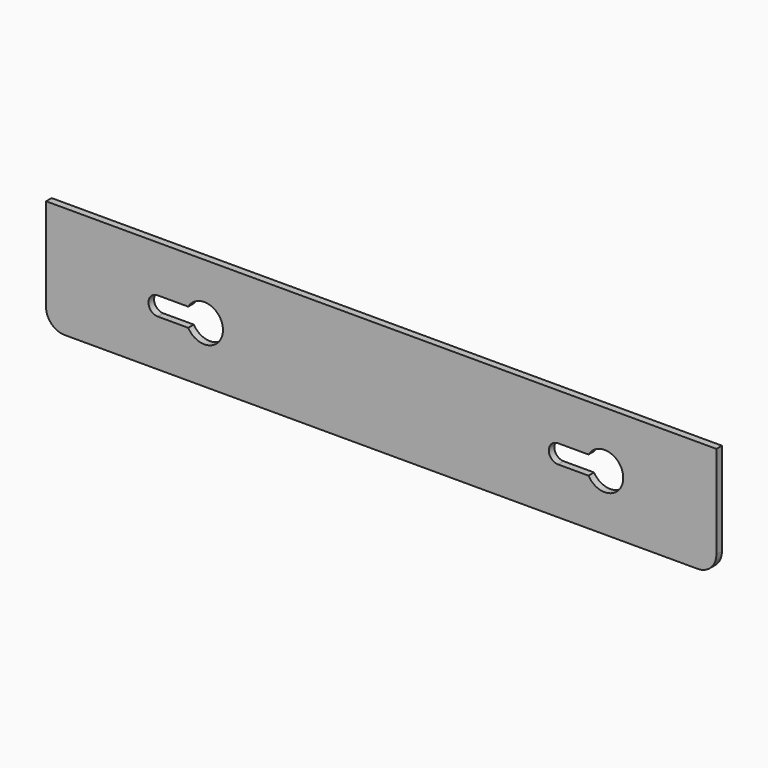
from build123d import *

# Parameters (mm, degrees)
F1_DEPTH = 4.7498


# Not quite as in the source:
# - a feature names something its author has since deleted; it is built from what else it names


with BuildPart() as f1:
    # F0 (on Front) → F1 (new body)
    with BuildSketch(Plane.XZ):
        with BuildLine():
            Line((304.8, -368.3), (304.8, -304.8))
            Line((304.8, -304.8), (0, -304.8))
            Line((0, -304.8), (-152.4, -304.8))
            Line((-152.4, -304.8), (-152.4, -368.3))
            ThreePointArc((-152.4, -368.3), (-148.6802561211, -377.2802561211), (-139.7, -381))
            Line((-139.7, -381), (292.1, -381))
            ThreePointArc((292.1, -381), (301.0802561211, -377.2802561211), (304.8, -368.3))
        make_face()
        with BuildLine():
            ThreePointArc((-55.4485226281, -336.55), (-31.75, -342.9), (-55.4485226281, -349.25))
            Line((-55.4485226281, -349.25), (-76.2, -349.25))
            ThreePointArc((-76.2, -349.25), (-82.55, -342.9), (-76.2, -336.55))
            Line((-76.2, -336.55), (-55.4485226281, -336.55))
        make_face(mode=Mode.SUBTRACT)
        with BuildLine():
            ThreePointArc((217.6014773719, -336.55), (241.3, -342.9), (217.6014773719, -349.25))
            Line((217.6014773719, -349.25), (196.85, -349.25))
            ThreePointArc((196.85, -349.25), (190.5, -342.9), (196.85, -336.55))
            Line((196.85, -336.55), (217.6014773719, -336.55))
        make_face(mode=Mode.SUBTRACT)
    extrude(amount=F1_DEPTH)


solid = f1.part
